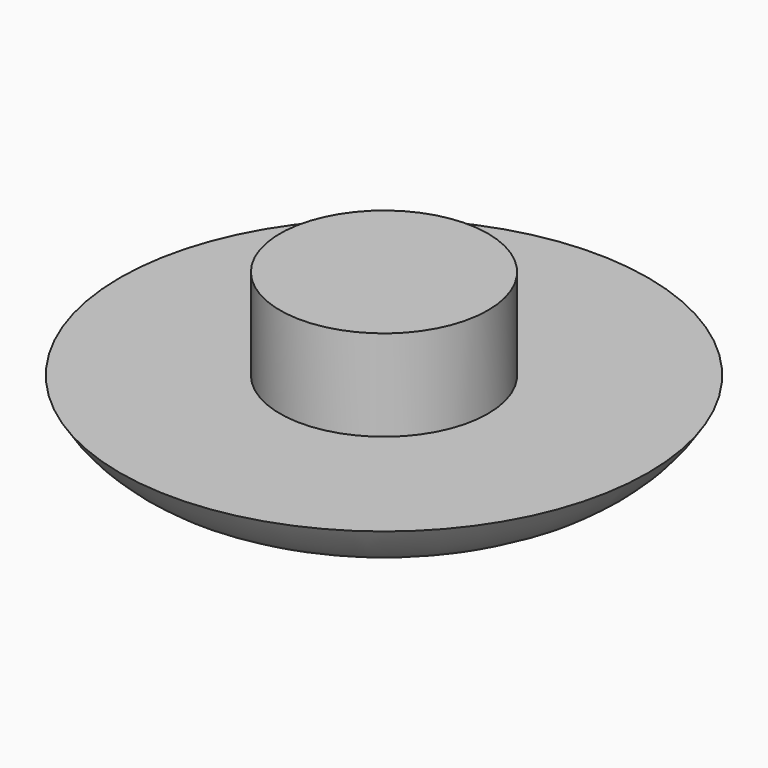
from build123d import *

# Parameters (mm, degrees)
F0_R     = 10.16
F1_DEPTH = 2.5
F2_R     = 4
F3_DEPTH = 3.5


# Not quite as in the source:
# - a fillet or chamfer that OpenCascade refuses, or shapes differently, is made with other operations: its cross-section is extruded or revolved along the edge and cut away or added


with BuildPart() as f1:
    # F0 (on Top) → F1 (new body)
    with BuildSketch(Plane.XY):
        Circle(F0_R)
    extrude(amount=F1_DEPTH)

    # F2 (on face) → F3 (join)
    with BuildSketch(Plane.XY.offset(2.5)):
        Circle(F2_R)
    extrude(amount=F3_DEPTH)

    # F4: fillet of radius 5 on 1 edges, made by hand

    # F4_s1 → F4_t2 (revolve, cut)
    with BuildSketch(Plane.XZ):
        with BuildLine():
            ThreePointArc((10.16, 2.5), (8.3298729811, 0.6698729811), (5.8298729811, 0))
            Line((5.8298729811, 0), (10.16, 0))
            Line((10.16, 0), (10.16, 2.5))
        make_face()
    revolve(axis=Axis((0, 0, 0), (0, 0, 1)), mode=Mode.SUBTRACT)

    # F5: F1 across plane


with BuildPart() as f1_1:
    add(f1.part)
    add(f1.part.mirror(Plane.XZ))


solid = f1_1.part
